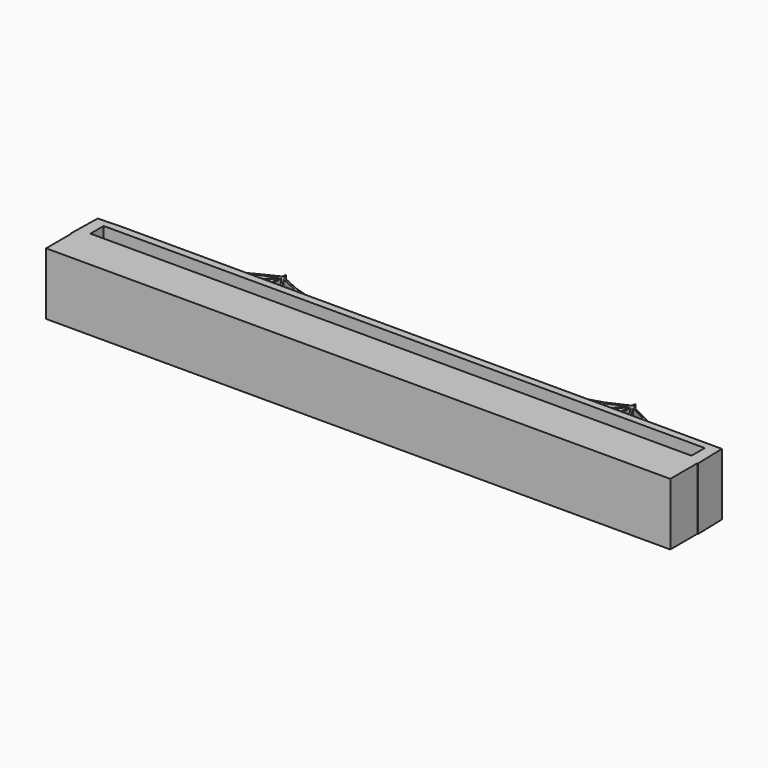
from build123d import *

# Parameters (mm, degrees)
F1_DEPTH = 3
F2_DEPTH = 6


# Not quite as in the source:
# - ends of sketch curves that miss each other by under 0.0002 mm in the source are joined


with BuildPart() as f1:
    # F0 (on Top) → F1 (new body)
    with BuildSketch(Plane.XY):
        Polygon((-28.9102834376, -0.4414349821), (-28.257415627, -0.4419910811), (-27.8283658653, -0.4208795241), (-21.8995697455, -0.158528512), (-17.4913680187, 0.0069514035), (-16.3024572399, 0.12255881), (-16.3007439351, 0.0480150165), (-5.6757512867, 0.2795930401), (-0.7151074092, 0.2985909701), (8.2958557755, 0.2619552836), (16.2606113526, 0.0699087279), (16.2623272719, 0.156866082), (17.4677160222, 0.126886716), (17.469259561, 0.0407657468), (18.1427192444, 0.024527256), (25.1678855365, -0.2592209701), (28.889729186, -0.4474497414), (28.8916880976, -0.3719352481), (30.0944449, -0.4916939621), (28.0635175414, 1.4387395664), (27.1957001251, 1.5829541625), (26.0534694908, 1.8402576865), (24.9059942644, 2.0530012286), (20.5818540671, 3.375628251), (16.9379126621, 5.2689424736), (16.76655207, 5.2689424736), (14.7802347314, 4.3726547053), (11.3282385864, 3.377332845), (8.6960734156, 2.8465205968), (7.4637700632, 2.6609695328), (5.7395421167, 2.4522244587), (2.3759140957, 2.2760017987), (0.7180276472, 2.2760017987), (-0.8097978472, 2.2760017987), (-0.9811586933, 2.2760017987), (-2.4124626637, 2.2665616347), (-4.1395994182, 2.3621735847), (-5.7662817127, 2.4522244587), (-6.640232213, 2.5329408328), (-7.4905099132, 2.6609695328), (-8.7228130116, 2.8465205968), (-9.949872026, 3.0866618489), (-11.2696873543, 3.3596889326), (-11.3379799944, 3.372315329), (-14.8069745814, 4.3726547053), (-16.793291666, 5.2689424736), (-16.9646525121, 5.2689424736), (-18.8665346626, 4.3341409393), (-20.6085936631, 3.375628251), (-22.3328218637, 2.8285716868), (-23.7056751001, 2.4082918567), (-24.9326411504, 2.0526806806), (-24.9496969742, 2.049518972), (-27.2224397211, 1.5829541625), (-28.0902571374, 1.4387395664), (-30.113040494, -0.5218498582), align=None)
        Polygon((-28.0902571374, -0.1719470781), (-29.5294175818, -0.2427615161), (-28.9578396036, 0.3288162081), align=None, mode=Mode.SUBTRACT)
        Polygon((-27.9188962913, -0.1719470781), (-27.9188962913, 0.5617141422), (-27.2259680351, -0.136923526), align=None, mode=Mode.SUBTRACT)
        Polygon((-27.0510788751, -0.140480796), (-27.0510788751, 0.5911537582), (-26.0802090868, -0.044246038), align=None, mode=Mode.SUBTRACT)
        Polygon((-28.0902571374, 1.1963989284), (-28.0902571374, 0.025909778), (-28.8323907816, 0.4542650301), align=None, mode=Mode.SUBTRACT)
        Polygon((-27.8387770713, 0.7242761742), (-27.2224397211, 1.3406132704), (-27.2224397211, 0.102860348), align=None, mode=Mode.SUBTRACT)
        Polygon((-26.948988909, 0.7291369722), (-26.0802090868, 1.5979167945), (-26.0802090868, 0.160551622), align=None, mode=Mode.SUBTRACT)
        Polygon((-25.9088482407, -0.044246038), (-25.9088482407, 0.7817563742), (-24.9327341144, -0.010288524), align=None, mode=Mode.SUBTRACT)
        Polygon((-24.3011486362, 0.011369294), (-24.7613732684, -0.010288524), (-24.7613732684, 1.1208298643), (-24.3011486362, 0.6499031962), align=None, mode=Mode.SUBTRACT)
        Polygon((-24.1297877902, 0.011369294), (-24.1297877902, 0.4745573441), (-23.7056751001, 0.040582088), align=None, mode=Mode.SUBTRACT)
        Polygon((-24.1203130822, 0.7100371882), (-23.7056751001, 1.1439309103), (-23.7056751001, 0.2857568581), align=None, mode=Mode.SUBTRACT)
        Polygon((-23.534314254, 0.040582088), (-23.534314254, 1.3198365784), (-23.0571765239, 0.8316031122), (-23.0571765239, 0.07220585), align=None, mode=Mode.SUBTRACT)
        Polygon((-22.8858156778, 0.07220585), (-22.8858156778, 0.6562575142), (-22.3328218637, 0.090403934), align=None, mode=Mode.SUBTRACT)
        Polygon((-21.2925666414, 0.10996549), (-21.2925666414, 0.6975027962), (-20.6085936631, 0.154254708), align=None, mode=Mode.SUBTRACT)
        Polygon((-19.5678139308, 0.2021359941), (-19.5678139308, 0.7838836242), (-18.8665346626, 0.2268895641), align=None, mode=Mode.SUBTRACT)
        Polygon((-22.1614610176, 0.090403934), (-22.1614610176, 1.3876258764), (-21.4639274874, 0.8336069182), (-21.4639274874, 0.10996549), align=None, mode=Mode.SUBTRACT)
        Polygon((-22.8633930658, 0.8784882103), (-22.3328218637, 1.4090594124), (-22.3328218637, 0.3355787041), align=None, mode=Mode.SUBTRACT)
        Polygon((-19.7391747769, 0.2021359941), (-20.4372330711, 0.154254708), (-20.4372330711, 1.4744232644), (-19.7391747769, 0.9199874923), align=None, mode=Mode.SUBTRACT)
        Polygon((-17.7362067223, 0.2734597021), (-17.7362067223, 1.0145864903), (-16.9646525121, 0.2919201681), align=None, mode=Mode.SUBTRACT)
        Polygon((-16.793291666, 0.2919201681), (-15.9293792458, 1.2142757024), (-15.9293792458, 0.3273460561), align=None, mode=Mode.SUBTRACT)
        Polygon((-27.4307712832, 1.3746226004), (-27.9188962913, 0.8864975923), (-27.9188962913, 1.2935056684), align=None, mode=Mode.SUBTRACT)
        Polygon((-26.3069376148, 1.6135291585), (-27.0510788751, 0.8693876443), (-27.0510788751, 1.4459008424), align=None, mode=Mode.SUBTRACT)
        Polygon((-25.8161656727, 0.9272287783), (-24.9327341144, 1.8106605905), (-24.9327341144, 0.2103889621), align=None, mode=Mode.SUBTRACT)
        Polygon((-25.9088482407, 1.0768871023), (-25.9088482407, 1.6977471765), (-25.1466813625, 1.8390539805), align=None, mode=Mode.SUBTRACT)
        Polygon((-24.6349671203, 1.2366591984), (-23.7056751001, 2.1659509646), (-23.7056751001, 1.3919629264), (-24.2401530762, 0.8326638162), align=None, mode=Mode.SUBTRACT)
        Polygon((-24.7613732684, 1.3499904424), (-24.7613732684, 1.9242189106), (-23.9567815321, 2.1571854246), align=None, mode=Mode.SUBTRACT)
        Polygon((-22.9831708299, 1.0010510843), (-23.413465626, 1.4413522104), (-22.3328218637, 2.5805399248), (-22.3328218637, 1.6514000505), align=None, mode=Mode.SUBTRACT)
        Polygon((-22.5748993577, 2.5752521528), (-23.534314254, 1.5712815925), (-23.534314254, 2.2815407767), align=None, mode=Mode.SUBTRACT)
        Polygon((-21.2915818834, 0.9162785843), (-20.6085936631, 1.7999621105), (-20.6085936631, 0.3730896781), align=None, mode=Mode.SUBTRACT)
        Polygon((-19.5678139308, 1.0097477903), (-18.8665346626, 2.0732935426), (-18.8665346626, 0.4457247881), align=None, mode=Mode.SUBTRACT)
        Polygon((-17.9075675683, 0.2734597021), (-18.6951738166, 0.2268895641), (-18.6951738166, 1.9127906886), (-17.9075675683, 1.1734490123), align=None, mode=Mode.SUBTRACT)
        Polygon((-15.7580183997, 1.3972288544), (-14.9783354275, 2.2296569587), (-14.9783354275, 0.3459375861), (-15.7580183997, 0.3273460561), align=None, mode=Mode.SUBTRACT)
        Polygon((-17.7411096843, 1.2539672664), (-16.9646525121, 2.3454967067), (-16.9646525121, 0.5267088782), align=None, mode=Mode.SUBTRACT)
        Polygon((-16.793291666, 0.5425920062), (-16.793291666, 2.3756495547), (-15.9476448938, 1.4454461824), align=None, mode=Mode.SUBTRACT)
        Polygon((-22.1469477116, 1.5949335645), (-20.6085936631, 3.1332876129), (-20.6085936631, 2.0801799906), (-21.4271668294, 1.0210703483), align=None, mode=Mode.SUBTRACT)
        Polygon((-20.8719200352, 3.1123021329), (-22.1614610176, 1.8227608965), (-22.1614610176, 2.7031614728), align=None, mode=Mode.SUBTRACT)
        Polygon((-18.6103934426, 2.4617522527), (-17.0813523041, 2.4770692147), (-17.8673154263, 1.3721765804), (-18.7403571146, 2.1898998627), (-18.6951738166, 2.3331759287), align=None, mode=Mode.SUBTRACT)
        Polygon((-15.8301231577, 1.5709183725), (-16.640622426, 2.4624596427), (-15.0065164735, 2.4788291807), (-14.9949162935, 2.4626262667), align=None, mode=Mode.SUBTRACT)
        Polygon((-14.8028529234, 0.3499581521), (-14.1324133192, 1.0039637023), (-14.1324133192, 0.4040454201), align=None, mode=Mode.SUBTRACT)
        Polygon((-13.0465600169, 0.4780963261), (-12.2964794747, 1.1204712163), (-12.2964794747, 0.4607935921), align=None, mode=Mode.SUBTRACT)
        Polygon((-10.7909429882, 0.4885489341), (-11.3549781824, 0.4780963261), (-10.7909429882, 1.0022304063), align=None, mode=Mode.SUBTRACT)
        Polygon((-9.4112718838, 0.5053967542), (-9.9469154618, 0.5124699665), (-9.4112718838, 1.0391528623), align=None, mode=Mode.SUBTRACT)
        Polygon((-5.9376425588, 0.5285257402), (-7.4900450932, 0.5277076062), (-6.671458719, 1.4096839984), align=None, mode=Mode.SUBTRACT)
        Polygon((-5.7652933987, 0.5261249322), (-4.9374207692, 1.3600506746), (-4.1395994182, 0.5525668402), align=None, mode=Mode.SUBTRACT)
        Polygon((-2.5762573578, 0.5505587162), (-3.966773688, 0.5541191962), (-3.25488135, 1.3085203704), align=None, mode=Mode.SUBTRACT)
        Polygon((-2.4035033217, 0.5515366162), (-1.6920551635, 1.2905183744), (-0.9769986813, 0.5475234162), align=None, mode=Mode.SUBTRACT)
        Polygon((-0.7570656692, 0.5473179302), (-0.045617511, 1.2862996884), (0.6694387172, 0.5433047302), align=None, mode=Mode.SUBTRACT)
        Polygon((-13.2179208629, 0.4780963261), (-13.9610524732, 0.4040454201), (-13.9610524732, 1.1711238963), (-13.2179208629, 1.8960398966), align=None, mode=Mode.SUBTRACT)
        Polygon((-12.1251186286, 1.2678646224), (-11.5263390284, 1.7828963585), (-11.5263390284, 0.4780963261), (-12.1251186286, 0.4607935921), align=None, mode=Mode.SUBTRACT)
        Polygon((-13.0465600169, 0.7013298142), (-13.0465600169, 2.0632003446), (-12.3732809467, 1.2804411784), align=None, mode=Mode.SUBTRACT)
        Polygon((-14.8069745814, 0.5853264902), (-14.8069745814, 2.2001119327), (-14.1324133192, 1.2578948684), align=None, mode=Mode.SUBTRACT)
        Polygon((-10.121232872, 0.5095628622), (-10.6195821422, 0.4885489341), (-10.6195821422, 1.1614688483), (-10.121232872, 1.6245634265), align=None, mode=Mode.SUBTRACT)
        Polygon((-11.3549781824, 0.7120224522), (-11.3549781824, 1.8045526525), (-10.8101801862, 1.2182800124), align=None, mode=Mode.SUBTRACT)
        Polygon((-9.949872026, 0.7521750262), (-9.949872026, 1.6921101545), (-9.4805003458, 1.2111271184), align=None, mode=Mode.SUBTRACT)
        Polygon((-8.8941738577, 0.5271315342), (-9.2399110378, 0.5053967542), (-9.2399110378, 1.2067095504), (-8.8941738577, 1.5447716125), align=None, mode=Mode.SUBTRACT)
        Polygon((-7.6618707593, 0.5271315342), (-8.7228130116, 0.5271315342), (-7.6618707593, 1.5238839225), align=None, mode=Mode.SUBTRACT)
        Polygon((-7.7820856573, 1.6460663045), (-8.7228130116, 0.7622555242), (-8.7228130116, 2.6021888528), align=None, mode=Mode.SUBTRACT)
        Polygon((-13.0465600169, 2.3259839187), (-13.0465600169, 3.6249112171), (-11.5366514284, 2.0000561986), (-12.2433665507, 1.3921851764), align=None, mode=Mode.SUBTRACT)
        Polygon((-9.949872026, 1.9374667886), (-9.949872026, 2.8443209568), (-8.8941738577, 1.7886230425), (-9.3579776038, 1.3309300284), align=None, mode=Mode.SUBTRACT)
        Polygon((-11.3549781824, 2.0562869726), (-11.3549781824, 3.1319762109), (-10.121232872, 1.8584895526), (-10.6846511002, 1.3349290044), align=None, mode=Mode.SUBTRACT)
        Polygon((-7.6618707593, 2.5134793527), (-7.6618707593, 1.7682156665), (-8.5226584715, 2.6430902188), align=None, mode=Mode.SUBTRACT)
        Polygon((-8.8941738577, 2.7054451868), (-8.8941738577, 2.0309636806), (-9.7327731459, 2.8695629689), align=None, mode=Mode.SUBTRACT)
        Polygon((-5.8463519107, 0.6866829042), (-6.553920727, 1.5363238265), (-5.8550321067, 2.2893332427), (-5.0447754085, 1.4735774444), align=None, mode=Mode.SUBTRACT)
        Polygon((-7.4905099132, 0.7791058842), (-7.4905099132, 2.3931915567), (-6.782026697, 1.5424525925), align=None, mode=Mode.SUBTRACT)
        Polygon((-4.0562170602, 0.7121446262), (-4.8023783824, 1.4714026964), (-4.0648360422, 2.1954357927), (-3.369570732, 1.4366181584), align=None, mode=Mode.SUBTRACT)
        Polygon((-3.1366042179, 1.4333133644), (-2.4793792177, 2.1086046226), (-1.8109683115, 1.4140779444), (-2.4889110757, 0.7098985042), align=None, mode=Mode.SUBTRACT)
        Polygon((-1.6375256815, 1.4140101264), (-0.9272604013, 2.1517632866), (-0.1738139152, 1.4087116107), (-0.9295684993, 0.6743161522), align=None, mode=Mode.SUBTRACT)
        Polygon((-6.664488705, 1.6690924205), (-7.3280621812, 2.4659038827), (-6.0678292428, 2.3119562607), align=None, mode=Mode.SUBTRACT)
        Polygon((-5.5889368807, 2.2717668567), (-4.2975744643, 2.2070921067), (-4.9224901565, 1.5936226705), align=None, mode=Mode.SUBTRACT)
        Polygon((-3.8066176101, 2.1816575627), (-2.7201127978, 2.1218550406), (-3.251293854, 1.5614111525), align=None, mode=Mode.SUBTRACT)
        Polygon((-1.1461347413, 2.1046409526), (-1.6920330655, 1.5376159245), (-2.2377363177, 2.1046409526), align=None, mode=Mode.SUBTRACT)
        Polygon((0.5003029111, 2.1004222666), (-0.045595413, 1.5333972385), (-0.5912989192, 2.1004222666), align=None, mode=Mode.SUBTRACT)
        Polygon((-20.4372330711, 2.0216769326), (-18.8665346626, 4.0539230592), (-18.8665346626, 2.3845867987), (-19.7391747769, 1.1021250503), (-20.4383374631, 1.6941355505), align=None, mode=Mode.SUBTRACT)
        Polygon((-19.1295514087, 3.9938373272), (-20.4372330711, 2.3018948127), (-20.4372330711, 3.274326955), align=None, mode=Mode.SUBTRACT)
        Polygon((-17.1509246821, 4.9864457055), (-18.6941600106, 2.6460064482), (-18.6951738166, 4.2274258873), align=None, mode=Mode.SUBTRACT)
        Polygon((-18.4966448765, 2.6342611788), (-16.9646525121, 4.9576494715), (-16.9646525121, 2.6411237508), align=None, mode=Mode.SUBTRACT)
        Polygon((-16.793291666, 2.6303945368), (-16.793291666, 4.9745701895), (-15.1283313175, 2.6489784468), align=None, mode=Mode.SUBTRACT)
        Polygon((-14.9783354275, 2.7338383228), (-16.5944680859, 4.9912285255), (-14.9783354275, 4.2619795393), align=None, mode=Mode.SUBTRACT)
        Polygon((-14.8069745814, 2.4944842167), (-14.8069745814, 4.1098708772), (-13.2179208629, 2.2624254987), (-13.2179208629, 2.1354288006), (-14.0021946312, 1.3703795304), align=None, mode=Mode.SUBTRACT)
        Polygon((-11.5263390284, 3.249243947), (-11.5263390284, 2.2406930047), (-12.8177753588, 3.6304438451), align=None, mode=Mode.SUBTRACT)
        Polygon((-10.121232872, 2.9471216149), (-10.121232872, 2.1130666406), (-11.1410212823, 3.1580828389), align=None, mode=Mode.SUBTRACT)
        Polygon((-13.2179208629, 3.7468949711), (-13.2179208629, 2.5252093268), (-14.6048596694, 4.1376744792), align=None, mode=Mode.SUBTRACT)
        Polygon((0.9502590853, 0.5475234162), (1.6653155675, 1.2905183744), (2.3767637257, 0.5515366162), align=None, mode=Mode.SUBTRACT)
        Polygon((3.228141754, 1.3085203704), (3.940034092, 0.5541191962), (2.5495177618, 0.5505587162), align=None, mode=Mode.SUBTRACT)
        Polygon((4.9077843185, 1.3613899624), (5.7385538027, 0.5261249322), (4.1128598222, 0.5525668402), align=None, mode=Mode.SUBTRACT)
        Polygon((6.644719123, 1.4096839984), (7.4633054972, 0.5277076062), (5.9109029628, 0.5285257402), align=None, mode=Mode.SUBTRACT)
        Polygon((9.3845322878, 1.0391528623), (9.9201758658, 0.5124699665), (9.3845322878, 0.5053967542), align=None, mode=Mode.SUBTRACT)
        Polygon((10.7642031382, 1.0022304063), (11.3282385864, 0.4780963261), (10.7642031382, 0.4885489341), align=None, mode=Mode.SUBTRACT)
        Polygon((12.2697398787, 0.4607935921), (12.2697398787, 1.1204712163), (13.0198204209, 0.4780963261), align=None, mode=Mode.SUBTRACT)
        Polygon((14.1056737232, 0.4040454201), (14.1056737232, 1.0039637023), (14.7761130734, 0.3499581521), align=None, mode=Mode.SUBTRACT)
        Polygon((0.0775240383, 1.4141014898), (0.8309705252, 2.1571529126), (1.5412358055, 1.4193997524), (0.8332786232, 0.6797057782), align=None, mode=Mode.SUBTRACT)
        Polygon((1.7842287155, 1.4140779444), (2.4526396217, 2.1086046226), (3.1098646219, 1.4333133644), (2.4621712257, 0.7098985042), align=None, mode=Mode.SUBTRACT)
        Polygon((4.0380964462, 2.1954357927), (4.7756387864, 1.4714026964), (4.0294772102, 0.7121446262), (3.342831136, 1.4366181584), align=None, mode=Mode.SUBTRACT)
        Polygon((5.8282925107, 2.2893332427), (6.5271811309, 1.5363238265), (5.8196123147, 0.6866829042), (5.0180355585, 1.4735774444), align=None, mode=Mode.SUBTRACT)
        Polygon((6.755287101, 1.5424525925), (7.4637700632, 2.3931915567), (7.4637700632, 0.7791058842), align=None, mode=Mode.SUBTRACT)
        Polygon((2.2109967217, 2.1046409526), (1.6652934695, 1.5376159245), (1.1193951453, 2.1046409526), align=None, mode=Mode.SUBTRACT)
        Polygon((3.224554258, 1.5614111525), (2.6933732018, 2.1218550406), (3.7798780141, 2.1816575627), align=None, mode=Mode.SUBTRACT)
        Polygon((4.8957505605, 1.5936226705), (4.2708348683, 2.2070921067), (5.5621972847, 2.2717668567), align=None, mode=Mode.SUBTRACT)
        Polygon((6.0410896468, 2.3119562607), (7.3013223312, 2.4659038827), (6.637749109, 1.6690924205), align=None, mode=Mode.SUBTRACT)
        Polygon((7.6351309093, 1.5238839225), (8.6960734156, 0.5271315342), (7.6351309093, 0.5271315342), align=None, mode=Mode.SUBTRACT)
        Polygon((9.2131714417, 1.2067095504), (9.2131714417, 0.5053967542), (8.8674342616, 0.5271315342), (8.8674342616, 1.5447716125), align=None, mode=Mode.SUBTRACT)
        Polygon((10.5928422922, 1.1614688483), (10.5928422922, 0.4885489341), (10.094493022, 0.5095628622), (10.094493022, 1.6245634265), align=None, mode=Mode.SUBTRACT)
        Polygon((9.4537607498, 1.2111271184), (9.92313243, 1.6921101545), (9.92313243, 0.7521750262), align=None, mode=Mode.SUBTRACT)
        Polygon((10.7834405902, 1.2182800124), (11.3282385864, 1.8045526525), (11.3282385864, 0.7120224522), align=None, mode=Mode.SUBTRACT)
        Polygon((8.6960734156, 2.6021888528), (8.6960734156, 0.7622555242), (7.7553460613, 1.6460663045), align=None, mode=Mode.SUBTRACT)
        Polygon((11.4995994324, 0.4780963261), (11.4995994324, 1.7828963585), (12.0983790326, 1.2678646224), (12.0983790326, 0.4607935921), align=None, mode=Mode.SUBTRACT)
        Polygon((12.3465413507, 1.2804411784), (13.0198204209, 2.0632003446), (13.0198204209, 0.7013298142), align=None, mode=Mode.SUBTRACT)
        Polygon((13.9343128772, 1.1711238963), (13.9343128772, 0.4040454201), (13.1911812669, 0.4780963261), (13.1911812669, 1.8960398966), align=None, mode=Mode.SUBTRACT)
        Polygon((14.1056737232, 1.2578948684), (14.7802347314, 2.2001119327), (14.7802347314, 0.5853264902), align=None, mode=Mode.SUBTRACT)
        Polygon((8.8674342616, 1.7886230425), (9.92313243, 2.8443209568), (9.92313243, 1.9374667886), (9.3312380078, 1.3309300284), align=None, mode=Mode.SUBTRACT)
        Polygon((8.4959186215, 2.6430902188), (7.6351309093, 1.7682156665), (7.6351309093, 2.5134793527), align=None, mode=Mode.SUBTRACT)
        Polygon((9.7060335499, 2.8695629689), (8.8674342616, 2.0309636806), (8.8674342616, 2.7054451868), align=None, mode=Mode.SUBTRACT)
        Polygon((10.094493022, 1.8584895526), (11.3282385864, 3.1319762109), (11.3282385864, 2.0562869726), (10.6579115042, 1.3349290044), align=None, mode=Mode.SUBTRACT)
        Polygon((11.5099115784, 2.0000561986), (13.0198204209, 3.6249112171), (13.0198204209, 2.3259839187), (12.2166267006, 1.3921851764), align=None, mode=Mode.SUBTRACT)
        Polygon((15.9026396497, 0.3273460561), (15.9026396497, 1.2142757024), (16.76655207, 0.2919201681), align=None, mode=Mode.SUBTRACT)
        Polygon((16.9379126621, 0.2919201681), (17.7094671263, 1.0145864903), (17.7094671263, 0.2734597021), align=None, mode=Mode.SUBTRACT)
        Polygon((18.8397950666, 0.2268895641), (19.5410743348, 0.7838836242), (19.5410743348, 0.2021359941), align=None, mode=Mode.SUBTRACT)
        Polygon((20.5818540671, 0.154254708), (21.2658267913, 0.6975027962), (21.2658267913, 0.10996549), align=None, mode=Mode.SUBTRACT)
        Polygon((22.3060822677, 0.090403934), (22.8590760818, 0.6562575142), (22.8590760818, 0.07220585), align=None, mode=Mode.SUBTRACT)
        Polygon((20.4104932211, 1.4744232644), (20.4104932211, 0.154254708), (19.7124351809, 0.2021359941), (19.7124351809, 0.9199874923), align=None, mode=Mode.SUBTRACT)
        Polygon((21.4371876374, 0.8336069182), (22.1347214216, 1.3876258764), (22.1347214216, 0.090403934), (21.4371876374, 0.10996549), align=None, mode=Mode.SUBTRACT)
        Polygon((22.3060822677, 0.3355787041), (22.3060822677, 1.4090594124), (22.8366534698, 0.8784882103), align=None, mode=Mode.SUBTRACT)
        Polygon((27.1992281851, -0.136923526), (27.8921566953, 0.5617141422), (27.8921566953, -0.1719470781), align=None, mode=Mode.SUBTRACT)
        Polygon((28.9311000076, 0.3288162081), (29.5026777318, -0.2427615161), (28.0635175414, -0.1719470781), align=None, mode=Mode.SUBTRACT)
        Polygon((23.6789355041, 0.040582088), (24.1030481942, 0.4745573441), (24.1030481942, 0.011369294), align=None, mode=Mode.SUBTRACT)
        Polygon((24.7346334184, 1.1208298643), (24.7346334184, -0.010288524), (24.2744090402, 0.011369294), (24.2744090402, 0.6499031962), align=None, mode=Mode.SUBTRACT)
        Polygon((24.9059942644, -0.010288524), (25.8821086447, 0.7817563742), (25.8821086447, -0.044246038), align=None, mode=Mode.SUBTRACT)
        Polygon((23.0304369279, 0.8316031122), (23.507574658, 1.3198365784), (23.507574658, 0.040582088), (23.0304369279, 0.07220585), align=None, mode=Mode.SUBTRACT)
        Polygon((23.6789355041, 0.2857568581), (23.6789355041, 1.1439309103), (24.0935734862, 0.7100371882), align=None, mode=Mode.SUBTRACT)
        Polygon((26.0534694908, -0.044246038), (27.0243392791, 0.5911537582), (27.0243392791, -0.140480796), align=None, mode=Mode.SUBTRACT)
        Polygon((27.1957001251, 0.102860348), (27.1957001251, 1.3406132704), (27.8120374753, 0.7242761742), align=None, mode=Mode.SUBTRACT)
        Polygon((26.0534694908, 0.160551622), (26.0534694908, 1.5979167945), (26.922249059, 0.7291369722), align=None, mode=Mode.SUBTRACT)
        Polygon((28.8056511856, 0.4542650301), (28.0635175414, 0.025909778), (28.0635175414, 1.1963989284), align=None, mode=Mode.SUBTRACT)
        Polygon((14.9515955775, 0.3459375861), (14.9515955775, 2.2296569587), (15.7312788037, 1.3972288544), (15.7312788037, 0.3273460561), align=None, mode=Mode.SUBTRACT)
        Polygon((18.6684342206, 1.9127906886), (18.6684342206, 0.2268895641), (17.8808279723, 0.2734597021), (17.8808279723, 1.1734490123), align=None, mode=Mode.SUBTRACT)
        Polygon((15.9209052977, 1.4454461824), (16.76655207, 2.3756495547), (16.76655207, 0.5425920062), align=None, mode=Mode.SUBTRACT)
        Polygon((16.9379126621, 0.5267088782), (16.9379126621, 2.3454967067), (17.7143698343, 1.2539672664), align=None, mode=Mode.SUBTRACT)
        Polygon((18.8397950666, 0.4457247881), (18.8397950666, 2.0732935426), (19.5410743348, 1.0097477903), align=None, mode=Mode.SUBTRACT)
        Polygon((20.5818540671, 0.3730896781), (20.5818540671, 1.7999621105), (21.2648422873, 0.9162785843), align=None, mode=Mode.SUBTRACT)
        Polygon((14.9797768775, 2.4788291807), (16.613882576, 2.4624596427), (15.8033835617, 1.5709183725), (14.9681766975, 2.4626262667), align=None, mode=Mode.SUBTRACT)
        Polygon((17.8405758303, 1.3721765804), (17.0546127081, 2.4770692147), (18.5836538465, 2.4617522527), (18.6684342206, 2.3331759287), (18.7136175186, 2.1898998627), align=None, mode=Mode.SUBTRACT)
        Polygon((20.5818540671, 2.0801799906), (20.5818540671, 3.1332876129), (22.1202078616, 1.5949335645), (21.4004269794, 1.0210703483), align=None, mode=Mode.SUBTRACT)
        Polygon((22.1347214216, 2.7031614728), (22.1347214216, 1.8227608965), (20.8451801852, 3.1123021329), align=None, mode=Mode.SUBTRACT)
        Polygon((24.9059942644, 0.2103889621), (24.9059942644, 1.8106605905), (25.7894260767, 0.9272287783), align=None, mode=Mode.SUBTRACT)
        Polygon((23.6789355041, 1.3919629264), (23.6789355041, 2.1659509646), (24.6082275243, 1.2366591984), (24.2134132262, 0.8326638162), align=None, mode=Mode.SUBTRACT)
        Polygon((23.9300419361, 2.1571854246), (24.7346334184, 1.9242189106), (24.7346334184, 1.3499904424), align=None, mode=Mode.SUBTRACT)
        Polygon((25.1199415125, 1.8390539805), (25.8821086447, 1.6977471765), (25.8821086447, 1.0768871023), align=None, mode=Mode.SUBTRACT)
        Polygon((27.8921566953, 1.2935056684), (27.8921566953, 0.8864975923), (27.4040316872, 1.3746226004), align=None, mode=Mode.SUBTRACT)
        Polygon((27.0243392791, 1.4459008424), (27.0243392791, 0.8693876443), (26.2801980188, 1.6135291585), align=None, mode=Mode.SUBTRACT)
        Polygon((22.3060822677, 2.5805399248), (23.38672603, 1.4413522104), (22.9564312338, 1.0010510843), (22.3060822677, 1.6514000505), align=None, mode=Mode.SUBTRACT)
        Polygon((23.507574658, 2.2815407767), (23.507574658, 1.5712815925), (22.5481597617, 2.5752521528), align=None, mode=Mode.SUBTRACT)
        Polygon((11.1142816863, 3.1580828389), (10.094493022, 2.1130666406), (10.094493022, 2.9471216149), align=None, mode=Mode.SUBTRACT)
        Polygon((13.1911812669, 2.2624254987), (14.7802347314, 4.1098708772), (14.7802347314, 2.4944842167), (13.9754550352, 1.3703795304), (13.1911812669, 2.1354288006), align=None, mode=Mode.SUBTRACT)
        Polygon((12.7910355088, 3.6304438451), (11.4995994324, 2.2406930047), (11.4995994324, 3.249243947), align=None, mode=Mode.SUBTRACT)
        Polygon((14.5781200733, 4.1376744792), (13.1911812669, 2.5252093268), (13.1911812669, 3.7468949711), align=None, mode=Mode.SUBTRACT)
        Polygon((18.8397950666, 2.3845867987), (18.8397950666, 4.0539230592), (20.4104932211, 2.0216769326), (20.4115976131, 1.6941355505), (19.7124351809, 1.1021250503), align=None, mode=Mode.SUBTRACT)
        Polygon((20.4104932211, 3.274326955), (20.4104932211, 2.3018948127), (19.1028115587, 3.9938373272), align=None, mode=Mode.SUBTRACT)
        Polygon((15.1015917215, 2.6489784468), (16.76655207, 4.9745701895), (16.76655207, 2.6303945368), align=None, mode=Mode.SUBTRACT)
        Polygon((14.9515955775, 4.2619795393), (16.5677284899, 4.9912285255), (14.9515955775, 2.7338383228), align=None, mode=Mode.SUBTRACT)
        Polygon((16.9379126621, 2.6411237508), (16.9379126621, 4.9576494715), (18.4699050265, 2.6342611788), align=None, mode=Mode.SUBTRACT)
        Polygon((18.6684342206, 4.2274258873), (18.6674204146, 2.6460064482), (17.1241850861, 4.9864457055), align=None, mode=Mode.SUBTRACT)
        Polygon((-16.886580024, 5.6424695397), (-16.9646525121, 5.2689424736), (-16.793291666, 5.2689424736), align=None)
        Polygon((16.76655207, 5.2689424736), (16.9379126621, 5.2689424736), (16.844624558, 5.6424695397), align=None)
        Polygon((-17.5052142962, 0.005605018), (-17.5160347955, -0.4511403622), (-16.2892473962, -0.4521853138), (-16.3007439351, 0.0480150165), (-16.5314003939, 0.042987722), (-17.4913680187, 0.0069514035), align=None)
        Polygon((-16.5314003939, 0.042987722), (-16.3007439351, 0.0480150165), (-16.3024572399, 0.12255881), (-17.4913680187, 0.0069514035), align=None)
    extrude(amount=F1_DEPTH)


with BuildPart() as f1b:
    # F0 (on Top) → F1, piece 2 (new body)
    with BuildSketch(Plane.XY):
        Polygon((-29, -1.1948061456), (-28.8961617397, -1.1948061456), (-28.9096714128, -0.4740855756), (-29.2675263097, -0.4916939621), (-30.113040494, -0.5218498582), (-30.17472795, -3.7345028191), (-30.113040494, -3.7385855441), (-30.113040494, -1.9948061456), (-29, -1.9948061456), align=None)
    extrude(amount=F1_DEPTH)


with BuildPart() as f1c:
    # F0 (on Top) → F1, piece 3 (new body)
    with BuildSketch(Plane.XY):
        Polygon((16.2606113526, 0.0699087279), (16.249762015, -0.479901354), (17.4786101934, -0.4809480609), (17.469259561, 0.0407657468), align=None)
    extrude(amount=F1_DEPTH)


with BuildPart() as f1d:
    # F0 (on Top) → F1, piece 4 (new body)
    with BuildSketch(Plane.XY):
        Polygon((28.8886080964, -0.4906668559), (28.8703421108, -1.1948061456), (29, -1.1948061456), (29, -1.9948061456), (30.1155950874, -1.9948061456), (30.1155950874, -3.467762433), (30.17475335, -3.467762433), (30.0944449, -0.4916939621), (29.7645692579, -0.4916939621), (29.7589182489, -0.4914081676), align=None)
        Polygon((28.889729186, -0.4474497414), (28.8886080964, -0.4906668559), (29.7589182489, -0.4914081676), align=None)
    extrude(amount=F1_DEPTH)


with BuildPart() as f2:
    # F0 (on Top) → F2 (new body)
    with BuildSketch(Plane.XY):
        Polygon((28.8886080964, -0.4906668559), (28.8703421108, -1.1948061456), (29, -1.1948061456), (29, -1.9948061456), (30.1155950874, -1.9948061456), (30.1155950874, -3.467762433), (30.17475335, -3.467762433), (30.0944449, -0.4916939621), (29.7645692579, -0.4916939621), (29.7589182489, -0.4914081676), align=None)
        Polygon((29, -2.7948061456), (28.828836719, -2.7948061456), (28.8113796476, -3.467762433), (30.1155950874, -3.467762433), (30.1155950874, -1.9948061456), (29, -1.9948061456), align=None)
        Polygon((17.4786101934, -0.4809480609), (17.4914046113, -1.1948061456), (28.8703421108, -1.1948061456), (28.8886080964, -0.4906668559), align=None)
        Polygon((-16.1699545838, -5.6424695397), (-17.6377169523, -5.5874803177), (-17.5715572706, -2.7948061456), (-28.8661702591, -2.7948061456), (-28.8469086596, -3.8223832631), (-30.113040494, -3.7385855441), (-30.113040494, -6.7482306622), (30.1155950874, -6.7482306622), (30.1155950874, -3.467762433), (28.8113796476, -3.467762433), (28.828836719, -2.7948061456), (17.5200812757, -2.7948061456), (17.5321426142, -3.467762433), (16.1908029038, -3.467762433), (16.2040822711, -2.7948061456), (-16.2354049061, -2.7948061456), align=None)
        Polygon((16.249762015, -0.479901354), (16.2356548828, -1.1948061456), (17.4914046113, -1.1948061456), (17.4786101934, -0.4809480609), align=None)
        Polygon((17.5200812757, -2.7948061456), (16.2040822711, -2.7948061456), (16.1908029038, -3.467762433), (17.5321426142, -3.467762433), align=None)
        Polygon((-16.2892473962, -0.4521853138), (-16.2721790964, -1.1948061456), (16.2356548828, -1.1948061456), (16.249762015, -0.479901354), align=None)
        Polygon((-17.5160347955, -0.4511403622), (-17.5336525656, -1.1948061456), (-16.2721790964, -1.1948061456), (-16.2892473962, -0.4521853138), align=None)
        Polygon((-17.5715572706, -2.7948061456), (-17.6377169523, -5.5874803177), (-16.1699545838, -5.6424695397), (-16.2354049061, -2.7948061456), align=None)
        Polygon((-28.8961617397, -1.1948061456), (-17.5336525656, -1.1948061456), (-17.5160347955, -0.4511403622), (-28.257415627, -0.4419910811), (-28.9096714128, -0.4740855756), align=None)
        Polygon((-29, -1.1948061456), (-28.8961617397, -1.1948061456), (-28.9096714128, -0.4740855756), (-29.2675263097, -0.4916939621), (-30.113040494, -0.5218498582), (-30.17472795, -3.7345028191), (-30.113040494, -3.7385855441), (-30.113040494, -1.9948061456), (-29, -1.9948061456), align=None)
        Polygon((-28.8469086596, -3.8223832631), (-28.8661702591, -2.7948061456), (-29, -2.7948061456), (-29, -1.9948061456), (-30.113040494, -1.9948061456), (-30.113040494, -3.7385855441), align=None)
    extrude(amount=F2_DEPTH)


solid = Compound([f1.part, f1b.part, f1c.part, f1d.part, f2.part])
